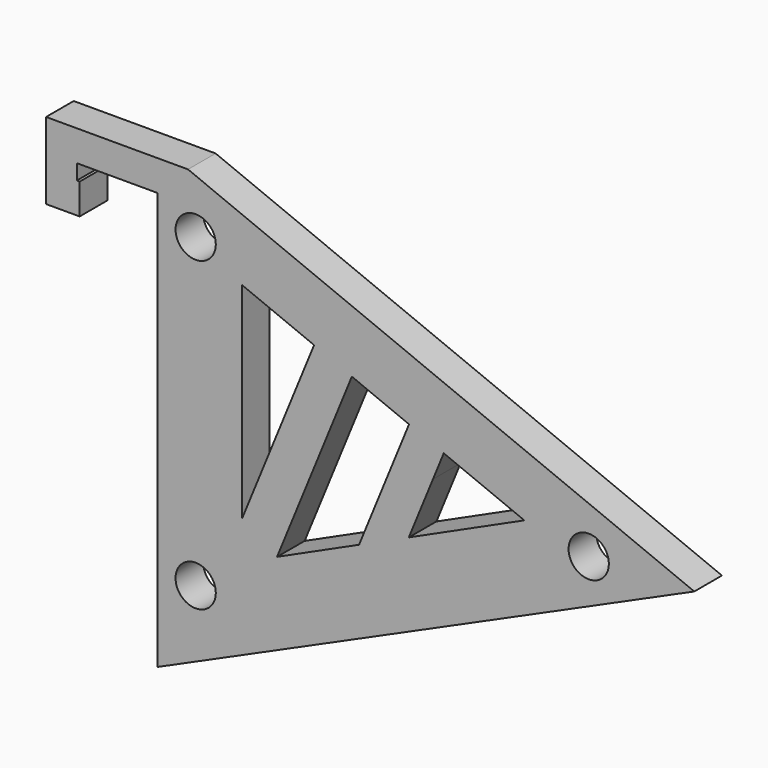
from build123d import *

# Parameters (mm, degrees)
F0_R     = 5.25
F0_W     = 0.75
F0_H     = 8
F1_DEPTH = 9


# Not quite as in the source:
# - a feature names something its author has since deleted; it is built from what else it names


with BuildPart() as f1:
    # F0 (on Front) → F1 (new body)
    with BuildSketch(Plane.XZ):
        Polygon((29, 0), (21, 0), (21, -8), (21, -109.6278309861), (21, -116.8163269758), (161, -53.9573058486), align=None)
        with Locations((31, -94.8660687473)):
            Circle(F0_R, mode=Mode.SUBTRACT)
        with Locations((31, -14.8660687473)):
            Circle(F0_R, mode=Mode.SUBTRACT)
        Polygon((43.1111576917, -75.528110744), (43.1111576917, -21.972979021), (61.8685626933, -29.6403959801), (71.7187130056, -33.6668169881), (86.6322777796, -39.7629971078), (95.6788662869, -43.460948191), (116.6788079217, -52.0450411727), (86.5560721122, -65.7548940175), (73.5966112911, -71.6531730426), (52.2128066716, -81.3856494169), (43.1111576917, -85.528110744), align=None, mode=Mode.SUBTRACT)
        with Locations((133.4695076596, -54.8660687473)):
            Circle(F0_R, mode=Mode.SUBTRACT)
        Polygon((71.7187130056, -33.6668169881), (61.8685626933, -29.6403959801), (43.1111576917, -75.528110744), (43.1111576917, -85.528110744), (52.2128066716, -81.3856494169), align=None)
        Polygon((21, -8), (21, 0), (-8, 0), (-8, -20), (0, -20), (0, -12), (0, -8), align=None)
        with Locations((0.375, -16)):
            Rectangle(F0_W, F0_H)
        Polygon((95.6788662869, -43.460948191), (86.6322777796, -39.7629971078), (73.5966112911, -71.6531730426), (86.5560721122, -65.7548940175), (86.6322777796, -65.5923289964), (92.8699112608, -50.3327157415), align=None)
    extrude(amount=F1_DEPTH)


solid = f1.part
